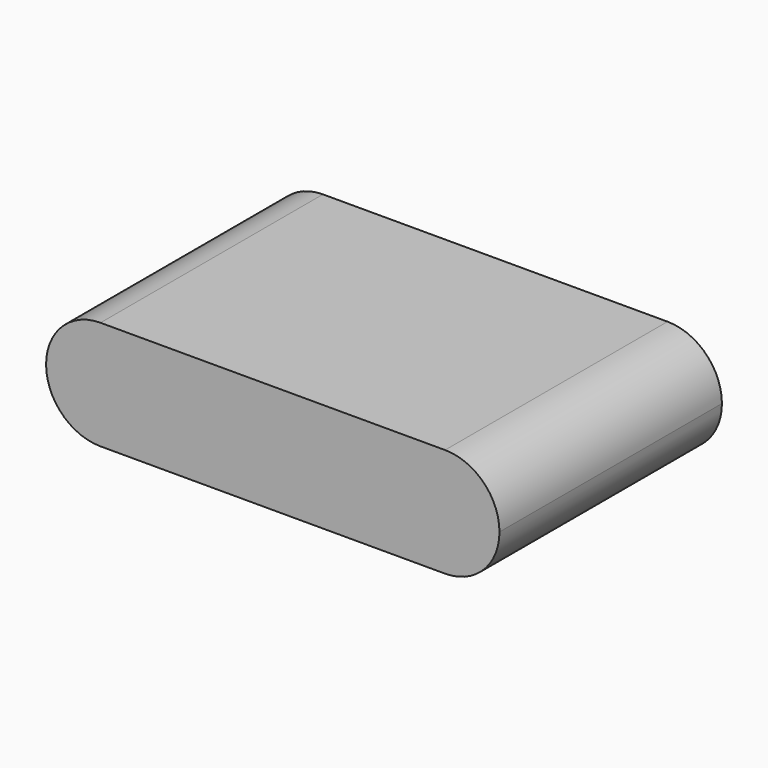
from build123d import *

# Parameters (mm, degrees)
F0_W     = 75
F0_H     = 46
F1_DEPTH = 18
F2_R     = 8.99999


# Not quite as in the source:
# - a fillet or chamfer is up to 0.001 mm smaller than in the source, because OpenCascade refuses the exact size


with BuildPart() as f1:
    # F0 (on Top) → F1 (new body)
    with BuildSketch(Plane.XY):
        Rectangle(F0_W, F0_H)
    extrude(amount=F1_DEPTH)

    # F2 (radius 9 in the source; OpenCascade refuses exactly that, so slightly less here)
    f2_edges = [f1.edges().sort_by_distance(p)[0] for p in [
        (37.5, 0, 18),
        (37.5, 0, 0),
        (-37.5, 0, 0),
        (-37.5, 0, 18),
    ]]
    fillet(f2_edges, radius=F2_R)


solid = f1.part
